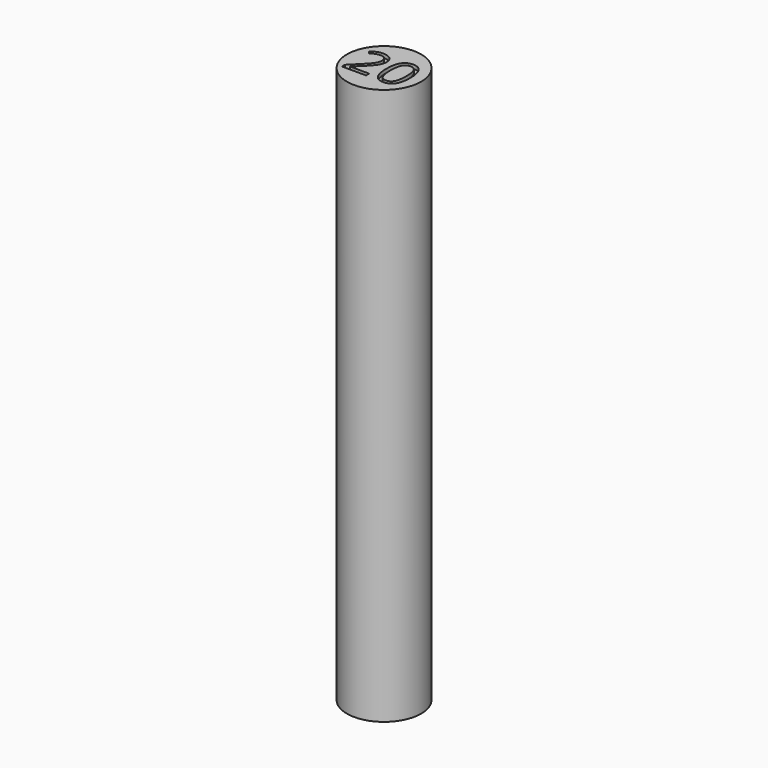
from build123d import *

# Parameters (mm, degrees)
F0_R         = 10
F1_DEPTH     = 150
F2_TEXT_SIZE = 13.8888888889
F3_DEPTH     = 1
F4_TEXT_SIZE = 13.8888888889
F5_DEPTH     = 1


# Not quite as in the source:
# - Text() gives the source's letters only with a copy of the font that has no kerning and outlines rounded to 1/6400 em; it was checked with that copy


with BuildPart() as f1:
    # F0 (on Top) → F1 (new body)
    with BuildSketch(Plane.XY):
        Circle(F0_R)
    extrude(amount=F1_DEPTH)

    # F2 (on face) → F3 (cut)
    with BuildSketch(Plane(origin=(0, 0, 0), x_dir=(1, 0, 0), z_dir=(0, 0, -1))):
        with Locations((-8.0457899306, -5)):
            Text('20', F2_TEXT_SIZE, font='Open Sans', text_align=(TextAlign.LEFT, TextAlign.BOTTOM))
    extrude(amount=-F3_DEPTH, mode=Mode.SUBTRACT)

    # F4 (on face) → F5 (cut)
    with BuildSketch(Plane.XY.offset(150)):
        with Locations((-8.0457899306, -5)):
            Text('20', F4_TEXT_SIZE, font='Open Sans', text_align=(TextAlign.LEFT, TextAlign.BOTTOM))
    extrude(amount=-F5_DEPTH, mode=Mode.SUBTRACT)


solid = f1.part
